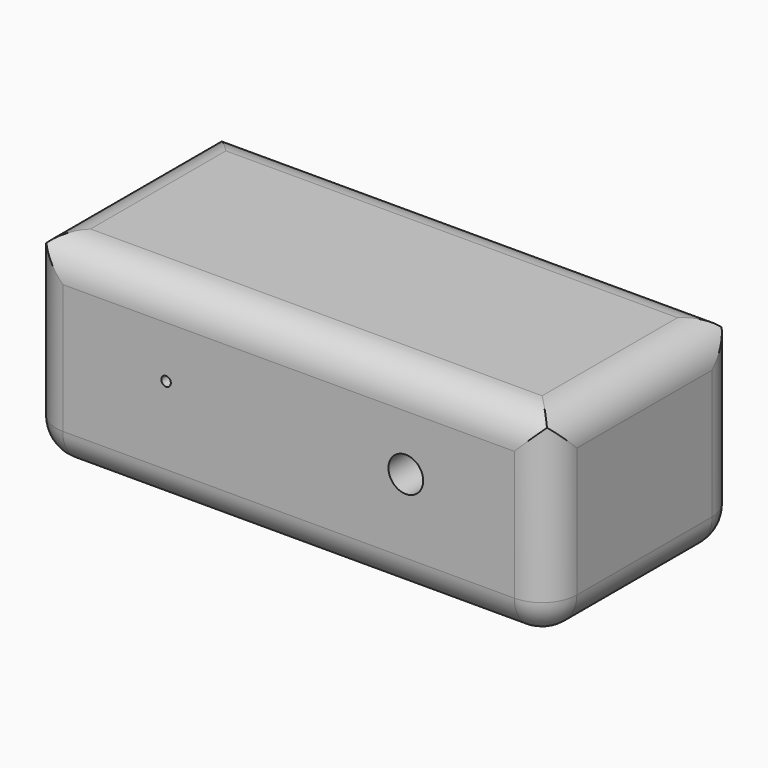
from build123d import *

# Parameters (mm, degrees)
F0_W           = 137.4083533883
F0_H           = 114.4303381443
F1_DEPTH       = 300
F2_R           = 20
F3_T1_DEPTH    = 124.4303381443
F3_T3_DEPTH    = 97.4083533883
F3_T5_DEPTH    = 260
F3_S9_W        = 20.4
F3_S9_H        = 20.4
F3_T10_DEPTH   = 20.4
F3_S15_W       = 20.4
F3_S15_H       = 20.4
F3_T16_DEPTH   = 20.4
F3_S21_W       = 20.4
F3_S21_H       = 20.4
F3_T22_DEPTH   = 20.4
F3_S27_W       = 20.4
F3_S27_H       = 20.4
F3_T28_DEPTH   = 20.4
F5_D           = 5.5
F7_D           = 20
F7_CSINK_D     = 25
F7_CSINK_ANGLE = 90


# Not quite as in the source:
# - a fillet or chamfer that OpenCascade refuses, or shapes differently, is made with other operations: its cross-section is extruded or revolved along the edge and cut away or added


with BuildPart() as f1:
    # F0 (on Right) → F1 (new body)
    with BuildSketch(Plane.YZ):
        with Locations((33.5574410856, 186.369523406)):
            Rectangle(F0_W, F0_H)
    extrude(amount=F1_DEPTH)

    # F2
    f2_edges = [f1.edges().sort_by_distance(p)[0] for p in [
        (150, 102.261618, 243.584692),
        (150, -35.146736, 243.584692),
        (0, 33.557441, 243.584692),
        (300, 33.557441, 243.584692),
    ]]
    fillet(f2_edges, radius=F2_R)

    # F3: fillet of radius 20 on 9 edges, made by hand

    # F3_s2 → F3_t1 (cut)
    with BuildSketch(Plane.XY.offset(149.1543543339)):
        with BuildLine():
            ThreePointArc((0, -15.1467356086), (5.8578643763, -29.2888712323), (20, -35.1467356086))
            Line((20, -35.1467356086), (0, -35.1467356086))
            Line((0, -35.1467356086), (0, -15.1467356086))
        make_face()
        with BuildLine():
            ThreePointArc((20, 102.2616177797), (5.8578643763, 96.4037534035), (0, 82.2616177797))
            Line((0, 82.2616177797), (0, 102.2616177797))
            Line((0, 102.2616177797), (20, 102.2616177797))
        make_face()
        with BuildLine():
            ThreePointArc((280, 102.2616177797), (294.1421356237, 96.4037534035), (300, 82.2616177797))
            Line((300, 82.2616177797), (300, 102.2616177797))
            Line((300, 102.2616177797), (280, 102.2616177797))
        make_face()
        with BuildLine():
            ThreePointArc((300, -15.1467356086), (294.1421356237, -29.2888712323), (280, -35.1467356086))
            Line((280, -35.1467356086), (300, -35.1467356086))
            Line((300, -35.1467356086), (300, -15.1467356086))
        make_face()
    extrude(amount=F3_T1_DEPTH, mode=Mode.SUBTRACT)

    # F3_s4 → F3_t3 (cut)
    with BuildSketch(Plane.XZ.offset(-82.2616177797)):
        with BuildLine():
            ThreePointArc((0, 149.1543543339), (5.8578643763, 135.0122187101), (20, 129.1543543339))
            Line((20, 129.1543543339), (0, 129.1543543339))
            Line((0, 129.1543543339), (0, 149.1543543339))
        make_face()
        with BuildLine():
            ThreePointArc((300, 149.1543543339), (294.1421356237, 135.0122187101), (280, 129.1543543339))
            Line((280, 129.1543543339), (300, 129.1543543339))
            Line((300, 129.1543543339), (300, 149.1543543339))
        make_face()
    extrude(amount=F3_T3_DEPTH, mode=Mode.SUBTRACT)

    # F3_s6 → F3_t5 (cut)
    with BuildSketch(Plane.YZ.offset(20)):
        with BuildLine():
            ThreePointArc((-35.1467356086, 149.1543543339), (-29.2888712323, 135.0122187101), (-15.1467356086, 129.1543543339))
            Line((-15.1467356086, 129.1543543339), (-35.1467356086, 129.1543543339))
            Line((-35.1467356086, 129.1543543339), (-35.1467356086, 149.1543543339))
        make_face()
        with BuildLine():
            ThreePointArc((102.2616177797, 149.1543543339), (96.4037534035, 135.0122187101), (82.2616177797, 129.1543543339))
            Line((82.2616177797, 129.1543543339), (102.2616177797, 129.1543543339))
            Line((102.2616177797, 129.1543543339), (102.2616177797, 149.1543543339))
        make_face()
    extrude(amount=F3_T5_DEPTH, mode=Mode.SUBTRACT)


with BuildPart() as f3_tool8:
    # F3_s9 → F3_t10 (new body)
    with BuildSketch(Plane.XZ.offset(15.1467356086)):
        with Locations((9.8, 138.9543543339)):
            Rectangle(F3_S9_W, F3_S9_H)
    extrude(amount=F3_T10_DEPTH)

    # F3_s11 → F3_t12 (revolve, cut)
    with BuildSketch(Plane(origin=(20, -15.1467356086, 149.1543543339), x_dir=(0.7071067812, 0, 0.7071067812), z_dir=(0.7071067812, 0, -0.7071067812))):
        with BuildLine():
            ThreePointArc((0, -20), (20, 0), (0, 20))
            Line((0, 20), (0, -20))
        make_face()
    revolve(axis=Axis((20, -15.1467356086, 149.1543543339), (0, -1, 0)), mode=Mode.SUBTRACT)


with BuildPart() as f1_1:
    add(f1.part)

    # F3_t7: cut F3_tool8
    add(f3_tool8.part, mode=Mode.SUBTRACT)


with BuildPart() as f3_tool14:
    # F3_s15 → F3_t16 (new body)
    with BuildSketch(Plane.XY.offset(149.1543543339)):
        with Locations((9.8, 92.4616177797)):
            Rectangle(F3_S15_W, F3_S15_H)
    extrude(amount=-F3_T16_DEPTH)

    # F3_s17 → F3_t18 (revolve, cut)
    with BuildSketch(Plane(origin=(20, 82.2616177797, 149.1543543339), x_dir=(0.7071067812, -0.7071067812, 0), z_dir=(0.7071067812, 0.7071067812, 0))):
        with BuildLine():
            ThreePointArc((0, -20), (20, 0), (0, 20))
            Line((0, 20), (0, -20))
        make_face()
    revolve(axis=Axis((20, 82.2616177797, 149.1543543339), (0, 0, -1)), mode=Mode.SUBTRACT)


with BuildPart() as f1_2:
    add(f1_1.part)

    # F3_t13: cut F3_tool14
    add(f3_tool14.part, mode=Mode.SUBTRACT)


with BuildPart() as f3_tool20:
    # F3_s21 → F3_t22 (new body)
    with BuildSketch(Plane.XZ.offset(15.1467356086)):
        with Locations((290.2, 138.9543543339)):
            Rectangle(F3_S21_W, F3_S21_H)
    extrude(amount=F3_T22_DEPTH)

    # F3_s23 → F3_t24 (revolve, cut)
    with BuildSketch(Plane(origin=(280, -15.1467356086, 149.1543543339), x_dir=(-0.7071067812, 0, 0.7071067812), z_dir=(0.7071067812, 0, 0.7071067812))):
        with BuildLine():
            ThreePointArc((0, -20), (20, 0), (0, 20))
            Line((0, 20), (0, -20))
        make_face()
    revolve(axis=Axis((280, -15.1467356086, 149.1543543339), (0, -1, 0)), mode=Mode.SUBTRACT)


with BuildPart() as f1_3:
    add(f1_2.part)

    # F3_t19: cut F3_tool20
    add(f3_tool20.part, mode=Mode.SUBTRACT)


with BuildPart() as f3_tool26:
    # F3_s27 → F3_t28 (new body)
    with BuildSketch(Plane.XY.offset(149.1543543339)):
        with Locations((290.2, 92.4616177797)):
            Rectangle(F3_S27_W, F3_S27_H)
    extrude(amount=-F3_T28_DEPTH)

    # F3_s29 → F3_t30 (revolve, cut)
    with BuildSketch(Plane(origin=(280, 82.2616177797, 149.1543543339), x_dir=(-0.7071067812, -0.7071067812, 0), z_dir=(0.7071067812, -0.7071067812, 0))):
        with BuildLine():
            ThreePointArc((0, -20), (20, 0), (0, 20))
            Line((0, 20), (0, -20))
        make_face()
    revolve(axis=Axis((280, 82.2616177797, 149.1543543339), (0, 0, -1)), mode=Mode.SUBTRACT)


with BuildPart() as f1_4:
    add(f1_3.part)

    # F3_t25: cut F3_tool26
    add(f3_tool26.part, mode=Mode.SUBTRACT)

    # F5 (through all)
    with Locations(Plane(origin=(0, 102.2616177797, 0), x_dir=(-1, 0, 0), z_dir=(0, 1, 0))):
        with Locations((-79.4825255871, 193.85394454)):
            Hole(F5_D / 2)

    # F7 (through all)
    with Locations(Plane(origin=(0, 102.2616177797, 0), x_dir=(-1, 0, 0), z_dir=(0, 1, 0))):
        with Locations((-217.5281494856, 191.5733516216)):
            CounterSinkHole(F7_D / 2, F7_CSINK_D / 2, counter_sink_angle=F7_CSINK_ANGLE)


solid = f1_4.part
